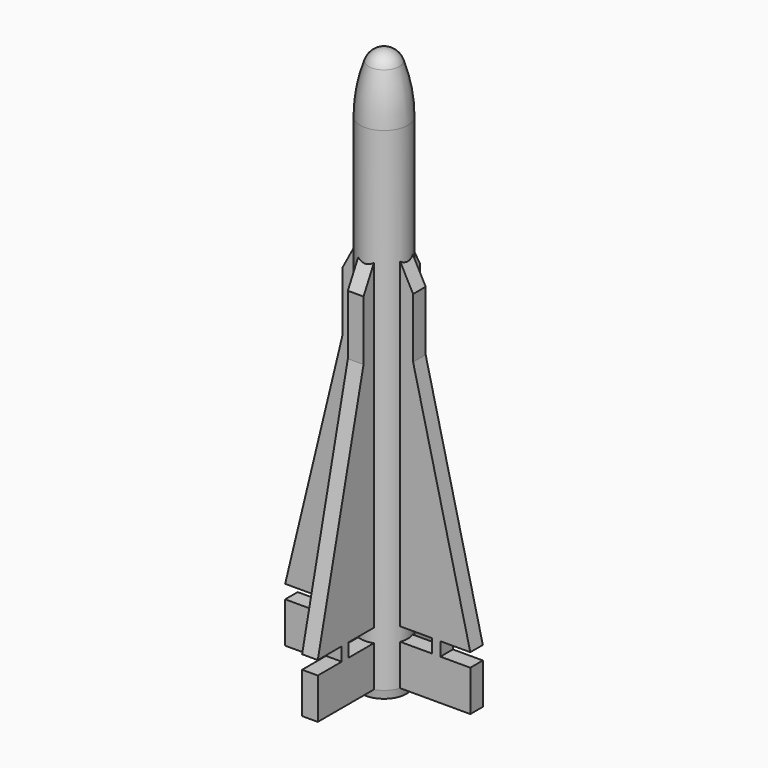
from build123d import *

# Parameters (mm, degrees)
F2_W     = 0.2083333333
F2_H     = 0.3472222222
F3_DEPTH = 0.2
F4_COUNT = 4


# Not quite as in the source:
# - a feature names something its author has since deleted; it is built from what else it names


with BuildPart() as f1:
    # F0 (on Front) → F1 (revolve)
    with BuildSketch(Plane.XZ):
        with BuildLine():
            Line((0, 14.3055555556), (0, 0))
            Line((0, 0), (0.5729166667, 0))
            Line((0.5729166667, 0), (0.6076388889, 0.2083333333))
            Line((0.6076388889, 0.2083333333), (0.6076388889, 12.7777777778))
            ThreePointArc((0.6076388889, 12.7777777778), (0.5535814562, 13.4119274316), (0.3929690636, 14.0277777778))
            ThreePointArc((0.3929690636, 14.0277777778), (0.2406164888, 14.2290996444), (0, 14.3055555556))
        make_face()
    revolve(axis=Axis((0, 0, 7.1527777778), (0, 0, 1)))

    # F2 (on Front) → F3 (join, symmetric)
    with BuildSketch(Plane.XZ):
        Polygon((0, 10.8660130719), (0, 0.2083333333), (0.6076388889, 0.2083333333), (2.3611111111, 0.2083333333), (2.3611111111, 1.25), (1.5972222222, 1.25), (1.3888888889, 1.25), (0.4, 1.25), (0.4, 1.5972222222), (1.3888888889, 1.5972222222), (1.5972222222, 1.5972222222), (2.3611111111, 1.5972222222), (0.9027777778, 7.6388888889), (0.9027777778, 9.1666666667), align=None)
        with Locations((1.4930555556, 1.4236111111)):
            Rectangle(F2_W, F2_H)
    extrude(amount=F3_DEPTH, both=True)

    # F4: F1 ×4 about axis
    f4_axis = Axis((0, 0, 0.2083333333), (0, 0, 1))


with BuildPart() as f1_1:
    add(f1.part)
    for i in range(1, F4_COUNT):
        add(f1.part.rotate(f4_axis, i * 360 / F4_COUNT))


solid = f1_1.part
